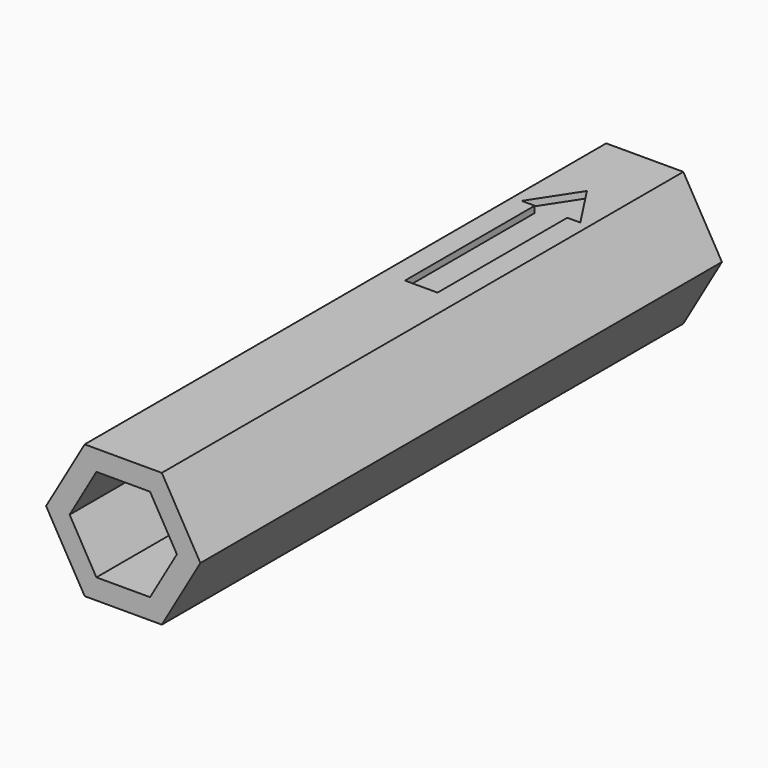
from build123d import *

# Parameters (mm, degrees)
F1_DEPTH     = 50.8
F3_DEPTH     = 25.4
F4_R         = 3.937
F5_DEPTH     = 25.4
F7_DEPTH     = 0.508
F8_TEXT_SIZE = 3.3157916208
F9_DEPTH     = 0.508


# Not quite as in the source:
# - Text() gives the source's letters only with a copy of the font that has no kerning and outlines rounded to 1/6400 em; it was checked with that copy


with BuildPart() as f1:
    # F0 (on Front) → F1 (new body)
    with BuildSketch(Plane.XZ):
        Polygon((3.0062628517, 5.207), (-3.0062628517, 5.207), (-6.0125257033, 0), (-3.0062628517, -5.207), (3.0062628517, -5.207), (6.0125257033, 0), align=None)
    extrude(amount=F1_DEPTH)

    # F2 (on face) → F3 (cut)
    with BuildSketch(Plane.XZ.offset(50.8)):
        Polygon((2.0897192993, 3.6195), (-2.0897192993, 3.6195), (-4.1794385987, 0), (-2.0897192993, -3.6195), (2.0897192993, -3.6195), (4.1794385987, 0), align=None)
    extrude(amount=-F3_DEPTH, mode=Mode.SUBTRACT)

    # F4 (on face) → F5 (cut)
    with BuildSketch(Plane(origin=(0, 0, 0), x_dir=(-1, 0, 0), z_dir=(0, 1, 0))):
        Circle(F4_R)
    extrude(amount=-F5_DEPTH, mode=Mode.SUBTRACT)

    # F6 (on face) → F7 (cut)
    with BuildSketch(Plane.XY.offset(5.207)):
        Polygon((2.286, -9.1356113553), (0, -5.634995643), (-2.286, -9.1356113553), (-1.27, -9.1356113553), (-1.27, -21.7719785869), (1.27, -21.7719785869), (1.27, -9.1356113553), align=None)
    extrude(amount=-F7_DEPTH, mode=Mode.SUBTRACT)

    # F8 (on face) → F9 (cut)
    with BuildSketch(Plane(origin=(0, 0, -5.207), x_dir=(1, 0, 0), z_dir=(0, 0, -1))):
        with Locations(Location((-0.9384654206, 37.957576348), (0, 0, -90))):
            Text('CHRIS JENTZSCH', F8_TEXT_SIZE, font='Open Sans', text_align=(TextAlign.LEFT, TextAlign.BOTTOM))
    extrude(amount=-F9_DEPTH, mode=Mode.SUBTRACT)


solid = f1.part
